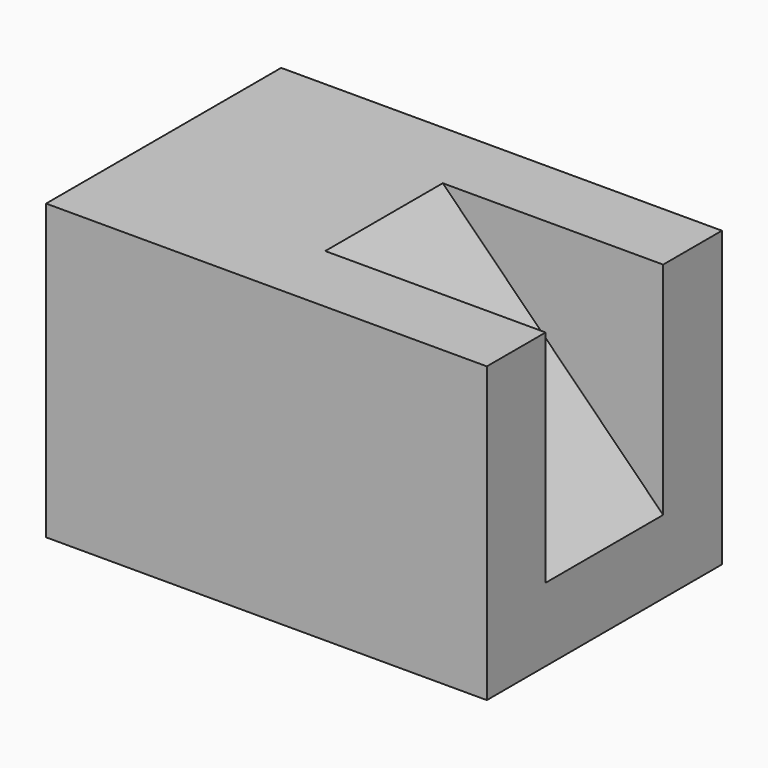
from build123d import *

# Parameters (mm, degrees)
F0_W     = 38.1
F0_H     = 25.4
F1_DEPTH = 12.7
F3_DEPTH = 6.35


# Not quite as in the source:
# - a feature names something its author has since deleted; it is built from what else it names


with BuildPart() as f1:
    # F0 (on Top) → F1 (new body, symmetric)
    with BuildSketch(Plane.XY):
        with Locations((19.05, 0)):
            Rectangle(F0_W, F0_H)
    extrude(amount=F1_DEPTH, both=True)

    # F2 (on Front) → F3 (cut, symmetric)
    with BuildSketch(Plane.XZ):
        Polygon((38.1, -6.35), (38.1, 12.7), (19.05, 12.7), align=None)
    extrude(amount=F3_DEPTH, both=True, mode=Mode.SUBTRACT)


solid = f1.part
